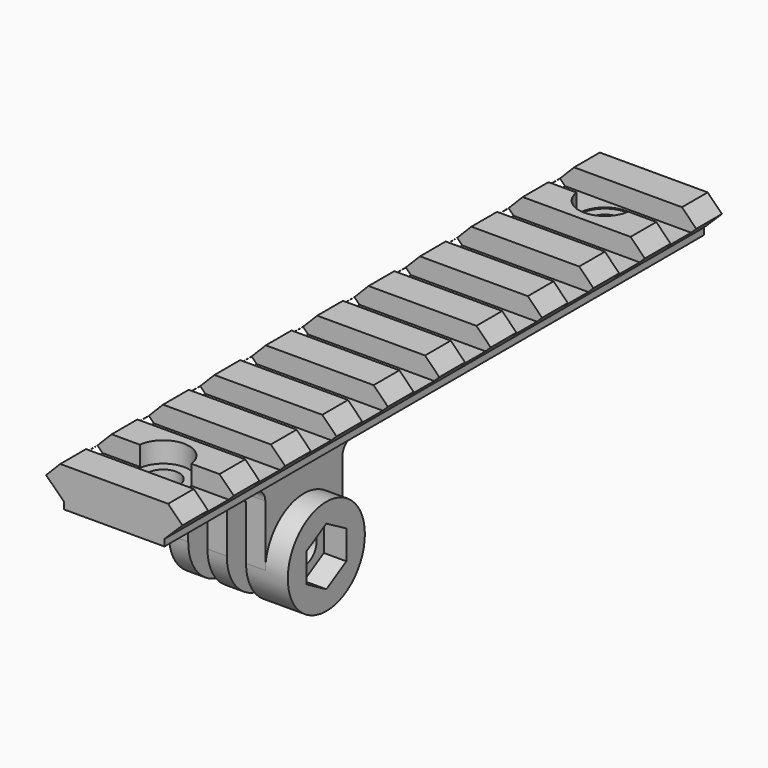
from build123d import *

# Parameters (mm, degrees)
F1_DEPTH       = 52.5
F2_W           = 21.2101023644
F2_H           = 4.993801238
F3_DEPTH       = 5
F5_D           = 5
F5_DEPTH       = 6.1
F5_CBORE_D     = 8.1
F5_CBORE_DEPTH = 3.2
F5_TIP         = 1.5021515476
F6_D           = 5
F6_DEPTH       = 6.1
F6_CBORE_D     = 8.1
F6_CBORE_DEPTH = 3.2
F6_TIP         = 1.5021515476
F7_R           = 2.5
F8_DEPTH       = 15
F9_DEPTH       = 18.5
F11_DEPTH      = 3.5
F13_START      = -3
F12_W          = 16
F12_H          = 15
F13_DEPTH      = 3
F14_START      = -9
F14_DEPTH      = 3
F15_ANGLE      = -90
F18_W          = 25
F18_H          = 18
F19_DEPTH      = 14
F21_R          = 2


with BuildPart() as f1:
    # F0 (on Front) → F1 (new body, symmetric)
    with BuildSketch(Plane.XZ):
        Polygon((-7.7991238795, -1.9758003764), (-7.7991238795, -3.0126834754), (7.814229466, -3.0126834754), (7.814229466, -1.9758003764), (10.6093045324, 0.7892206195), (8.3899200651, 3.0327284253), (-8.4017119181, 3.0327284253), (-10.6092272326, 0.7892206195), align=None)
    extrude(amount=F1_DEPTH, both=True)

    # F2 (on Top) → F3 (cut)
    with BuildSketch(Plane.XY):
        with Locations((0.0056419522, -4.9968052143)):
            Rectangle(F2_W, F2_H)
        with Locations((0.0056419522, -14.9968052143)):
            Rectangle(F2_W, F2_H)
        with Locations((0.0056419522, -24.9968052143)):
            Rectangle(F2_W, F2_H)
        with Locations((0.0056419522, -34.9968052143)):
            Rectangle(F2_W, F2_H)
        with Locations((0.0056419522, -44.9968052143)):
            Rectangle(F2_W, F2_H)
        with Locations((0.0056419522, 5.0031947857)):
            Rectangle(F2_W, F2_H)
        with Locations((0.0056419522, 15.0031947857)):
            Rectangle(F2_W, F2_H)
        with Locations((0.0056419522, 25.0031947857)):
            Rectangle(F2_W, F2_H)
        with Locations((0.0056419522, 35.0031947857)):
            Rectangle(F2_W, F2_H)
        with Locations((0.0056419522, 45.0031947857)):
            Rectangle(F2_W, F2_H)
    extrude(amount=F3_DEPTH, mode=Mode.SUBTRACT)

    # F5
    with Locations(Plane.XY.offset(3.0327284253)):
        with Locations((0, 42.9945960641)):
            CounterBoreHole(F5_D / 2, F5_CBORE_D / 2, F5_CBORE_DEPTH, depth=F5_DEPTH)
            with Locations((0, 0, -(F5_DEPTH + F5_TIP / 2))):  # 118° drill point
                Cone(0, F5_D / 2, F5_TIP, mode=Mode.SUBTRACT)

    # F6
    with Locations(Plane.XY.offset(3.0327284253)):
        with Locations((0, -42.977001518)):
            CounterBoreHole(F6_D / 2, F6_CBORE_D / 2, F6_CBORE_DEPTH, depth=F6_DEPTH)
            with Locations((0, 0, -(F6_DEPTH + F6_TIP / 2))):  # 118° drill point
                Cone(0, F6_D / 2, F6_TIP, mode=Mode.SUBTRACT)


with BuildPart() as f8:
    # F7 (on face) → F8 (new body)
    with BuildSketch(Plane(origin=(0, 0, -3.0126834754), x_dir=(1, 0, 0), z_dir=(0, 0, -1))):
        with BuildLine():
            ThreePointArc((-106.589045567, 38.187250495), (-108.7857447081, 43.4905513539), (-114.089045567, 45.687250495))
            ThreePointArc((-114.089045567, 45.687250495), (-119.3923464259, 43.4905513539), (-121.589045567, 38.187250495))
            ThreePointArc((-121.589045567, 38.187250495), (-119.3923464259, 32.8839496361), (-114.089045567, 30.687250495))
            ThreePointArc((-114.089045567, 30.687250495), (-108.7857447081, 32.8839496361), (-106.589045567, 38.187250495))
        make_face()
        with Locations((-114.089045567, 38.187250495)):
            Circle(F7_R, mode=Mode.SUBTRACT)
        with BuildLine():
            Line((-86.589045567, 45.687250495), (-114.089045567, 45.687250495))
            ThreePointArc((-114.089045567, 45.687250495), (-108.7857447081, 43.4905513539), (-106.589045567, 38.187250495))
            ThreePointArc((-106.589045567, 38.187250495), (-108.7857447081, 32.8839496361), (-114.089045567, 30.687250495))
            Line((-114.089045567, 30.687250495), (-86.589045567, 30.687250495))
            Line((-86.589045567, 30.687250495), (-86.589045567, 45.687250495))
        make_face()
    extrude(amount=F8_DEPTH)

    # F7 (on face) → F9 (join)
    with BuildSketch(Plane(origin=(0, 0, -3.0126834754), x_dir=(1, 0, 0), z_dir=(0, 0, -1))):
        with BuildLine():
            ThreePointArc((-106.589045567, 38.187250495), (-108.7857447081, 43.4905513539), (-114.089045567, 45.687250495))
            ThreePointArc((-114.089045567, 45.687250495), (-119.3923464259, 43.4905513539), (-121.589045567, 38.187250495))
            ThreePointArc((-121.589045567, 38.187250495), (-119.3923464259, 32.8839496361), (-114.089045567, 30.687250495))
            ThreePointArc((-114.089045567, 30.687250495), (-108.7857447081, 32.8839496361), (-106.589045567, 38.187250495))
        make_face()
        with Locations((-114.089045567, 38.187250495)):
            Circle(F7_R, mode=Mode.SUBTRACT)
    extrude(amount=F9_DEPTH)

    # F10 (on face) → F11 (cut)
    with BuildSketch(Plane(origin=(0, 0, -21.5126834754), x_dir=(1, 0, 0), z_dir=(0, 0, -1))):
        Polygon((-111.839045567, 34.2901361779), (-109.589045567, 38.187250495), (-111.839045567, 42.084364812), (-116.339045567, 42.084364812), (-118.589045567, 38.187250495), (-116.339045567, 34.2901361779), align=None)
    extrude(amount=-F11_DEPTH, mode=Mode.SUBTRACT)

    # F12 (on face) → F13 (cut)
    with BuildSketch(Plane.XY.offset(-3.0126834754).offset(F13_START)):
        with Locations((-113.6591356158, -38.187250793)):
            Rectangle(F12_W, F12_H)
    extrude(amount=-F13_DEPTH, mode=Mode.SUBTRACT)

    # F12 (on face) → F14 (cut)
    with BuildSketch(Plane.XY.offset(-3.0126834754).offset(F14_START)):
        with Locations((-113.6591356158, -38.187250793)):
            Rectangle(F12_W, F12_H)
    extrude(amount=-F14_DEPTH, mode=Mode.SUBTRACT)


with BuildPart() as f8_1:
    # F15: moved
    add(f8.part.rotate(Axis((-86.589045567, -38.187250495, -18.0126834754), (0, 1, 0)), F15_ANGLE))


with BuildPart() as f8_2:
    # F16: moved
    add(f8_1.part.moved(Location((94.1, 0, 31))))


with BuildPart() as f8_3:
    # F17: moved
    add(f8_2.part.moved(Location((0, 13.2, 0))))

    # F18 (on face) → F19 (cut)
    with BuildSketch(Plane.XY.offset(12.9873165246)):
        with Locations((0.6974760443, -24.6108990014)):
            Rectangle(F18_W, F18_H)
    extrude(amount=-F19_DEPTH, mode=Mode.SUBTRACT)


with BuildPart() as f1_1:
    add(f1.part)

    # F20: union F8
    add(f8_3.part)

    # F21
    f21_edges = [f1_1.edges().sort_by_distance(p)[0] for p in [
        (0.010954, -32.48725, -3.012683),
        (0.010954, -17.48725, -3.012683),
    ]]
    fillet(f21_edges, radius=F21_R)


solid = f1_1.part
